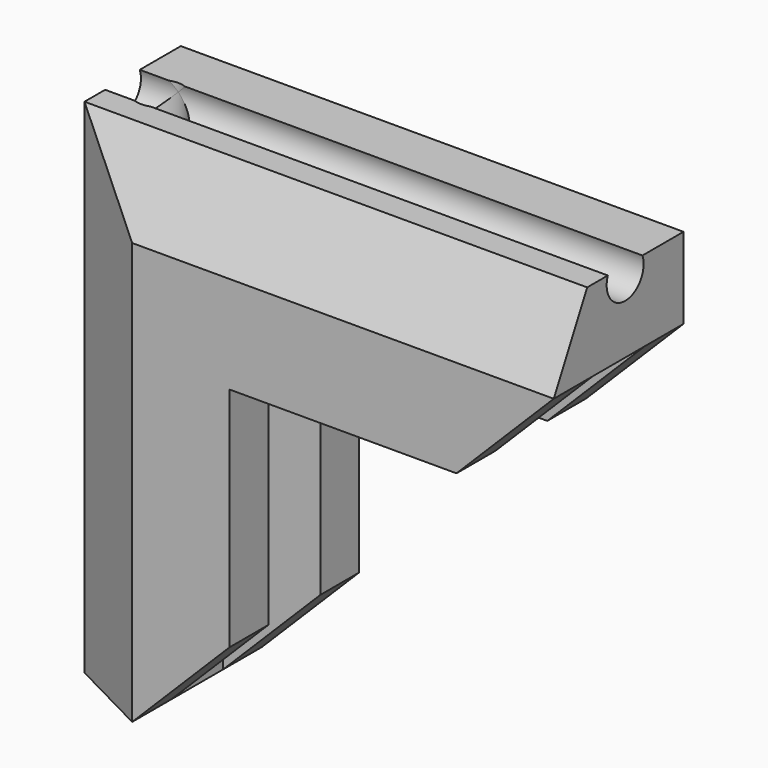
from build123d import *

# Parameters (mm, degrees)
F1_DEPTH      = 20
F2_W          = 7
F2_H          = 20
F3_DEPTH      = 2
F5_DEPTH      = 6
F6_W          = 3
F6_H          = 6
F7_DEPTH      = 25
F8_DEPTH      = 3
F12_DEPTH     = 2
F13_DEPTH     = 11
F14_T4_DEPTH  = 29
F14_T10_DEPTH = 28
F14_T17_DEPTH = 38.2867319519
F14_T24_DEPTH = 39.2867319519
F15_T1_DEPTH  = 61.1449358039
F15_T3_DEPTH  = 60.1449358039
F16_DEPTH     = 1
F17_SIZE      = 6
F20_D         = 2.85
F20_ON_F18_D  = 2.85
F22_DEPTH     = 3
F24_D         = 6.5
F24_DEPTH     = 2
F24_TIP       = 1.9527970118


# Not quite as in the source:
# - a fillet or chamfer that OpenCascade refuses, or shapes differently, is made with other operations: its cross-section is extruded or revolved along the edge and cut away or added


with BuildPart() as f1:
    # F0 (on Top) → F1 (new body)
    with BuildSketch(Plane.XY):
        Polygon((-3.1551690071, 9.1141472052), (-12.1551690071, 9.1141472052), (-12.1551690071, -0.8858527948), (-3.1551690071, -0.8858527948), (-3.1551690071, 2.1141472052), (-9.1551690071, 2.1141472052), (-9.1551690071, 6.1141472052), (-3.1551690071, 6.1141472052), align=None)
    extrude(amount=F1_DEPTH)

    # F2 (on face) → F3 (join)
    with BuildSketch(Plane(origin=(-12.1551690071, 0, 0), x_dir=(0, -1, 0), z_dir=(-1, 0, 0))):
        with Locations((-5.6141472052, 10)):
            Rectangle(F2_W, F2_H)
    extrude(amount=F3_DEPTH)

    # F4 (on face) → F5 (join)
    with BuildSketch(Plane.XY.offset(20)):
        Polygon((-12.1345976368, 9.1141472052), (-12.1551690071, 2.1141472052), (-12.1551690071, -0.8858527948), (-9.1551690071, -0.8858527948), (-9.1551690071, 2.1141472052), (-9.1551690071, 6.1141472052), (-9.1551690071, 9.1141472052), align=None)
    extrude(amount=F5_DEPTH)

    # F6 (on face) → F7 (join)
    with BuildSketch(Plane.YZ.offset(-9.1551690071)):
        with Locations((7.6141472052, 23)):
            Rectangle(F6_W, F6_H)
        with Locations((0.6141472052, 23)):
            Rectangle(F6_W, F6_H)
        Polygon((-0.8858527948, 26), (2.1141472052, 26), (6.1141472052, 26), (9.1141472052, 26), (9.1141472052, 29), (-0.8858527948, 29), align=None)
    extrude(amount=F7_DEPTH)

    # F8 (add): a face of the model
    f8_faces = [f1.faces().sort_by_distance(p)[0] for p in [
        (-10.6515768532, 4.1077318265, 26),
    ]]
    extrude(f8_faces, amount=F8_DEPTH)

    # F9: union 

    # F10: union 

    # F11 (on face) → F12 (join)
    with BuildSketch(Plane.XY.offset(29)):
        Polygon((-12.1345976368, 9.1141472052), (-12.1551690071, 2.1141472052), (15.8448309929, 2.1141472052), (15.8448309929, 9.1141472052), align=None)
    extrude(amount=F12_DEPTH)

    # F4 (on face) → F13 (join)
    with BuildSketch(Plane.XY.offset(20)):
        Polygon((-14.1551690071, 2.1141472052), (-12.1551690071, 2.1141472052), (-12.1345976368, 9.1141472052), (-14.1551690071, 9.1141472052), align=None)
    extrude(amount=F13_DEPTH)

    # F14: chamfer of 4 on 2 edges, made by hand


with BuildPart() as f14_tool2:
    # F14_s3 → F14_t4 (new body)
    with BuildSketch(Plane.XY):
        Polygon((-12.1551690071, -1.8858527948), (-16.1551690071, 2.1141472052), (-12.1551690071, 2.1141472052), align=None)
    extrude(amount=F14_T4_DEPTH)

    split(bisect_by=Plane.XZ.offset(0.8858527948), keep=Keep.BOTTOM)

    split(bisect_by=Plane.YZ.offset(-14.1551690071), keep=Keep.TOP)


with BuildPart() as f1_1:
    add(f1.part)

    # F14_t1: union F14_tool2
    add(f14_tool2.part)


with BuildPart() as f14_tool8:
    # F14_s9 → F14_t10 (new body)
    with BuildSketch(Plane.YZ.offset(-12.1551690071)):
        Polygon((-1.8858527948, 29), (2.1141472052, 33), (2.1141472052, 29), align=None)
    extrude(amount=F14_T10_DEPTH)

    split(bisect_by=Plane.XZ.offset(0.8858527948), keep=Keep.BOTTOM)

    split(bisect_by=Plane.XY.offset(31), keep=Keep.BOTTOM)


with BuildPart() as f1_2:
    add(f1_1.part)

    # F14_t7: union F14_tool8
    add(f14_tool8.part)


with BuildPart() as f14_tool15:
    # F14_s16 → F14_t17 (new body)
    with BuildSketch(Plane.YZ.offset(-22.4419009589)):
        Polygon((-1.8858527948, 29), (2.1141472052, 33), (2.1141472052, 29), align=None)
    extrude(amount=F14_T17_DEPTH)

    split(bisect_by=Plane.XZ.offset(0.8858527948), keep=Keep.BOTTOM)

    split(bisect_by=Plane.YZ.offset(-12.1551690071), keep=Keep.BOTTOM)

    split(bisect_by=Plane.YZ.offset(-14.1551690071), keep=Keep.TOP)

    split(bisect_by=Plane.XY.offset(31), keep=Keep.BOTTOM)


with BuildPart() as f14_tool22:
    # F14_s23 → F14_t24 (new body)
    with BuildSketch(Plane.XY):
        Polygon((-12.1551690071, -1.8858527948), (-16.1551690071, 2.1141472052), (-12.1551690071, 2.1141472052), align=None)
    extrude(amount=F14_T24_DEPTH)

    split(bisect_by=Plane.XZ.offset(0.8858527948), keep=Keep.BOTTOM)

    split(bisect_by=Plane.XY.offset(29), keep=Keep.TOP)

    split(bisect_by=Plane.YZ.offset(-14.1551690071), keep=Keep.TOP)

    split(bisect_by=Plane.XY.offset(31), keep=Keep.BOTTOM)


with BuildPart() as f14_tool15_1:
    add(f14_tool15.part)

    # F14_t29: intersect F14_tool22
    add(f14_tool22.part, mode=Mode.INTERSECT)


with BuildPart() as f1_3:
    add(f1_2.part)

    # F14_t13: union F14_tool15
    add(f14_tool15_1.part)

    # F15: chamfer of 4 x 6 on 2 edges, made by hand

    # F15_s2 → F15_t1 (cut)
    with BuildSketch(Plane.XY.offset(-15.5724679019)):
        Polygon((-9.1551690071, -0.8858527948), (-17.3978096942, 3.3567878923), (-13.1551690071, -0.8858527948), align=None)
    extrude(amount=F15_T1_DEPTH, mode=Mode.SUBTRACT)

    # F15_s4 → F15_t3 (cut)
    with BuildSketch(Plane.YZ.offset(-28.7276369091)):
        Polygon((-0.8858527948, 26), (3.3567878923, 34.2426406871), (-0.8858527948, 30), align=None)
    extrude(amount=F15_T3_DEPTH, mode=Mode.SUBTRACT)

    # F16 (add): a face of the model
    f16_faces = [f1_3.faces().sort_by_distance(p)[0] for p in [
        (15.8448309929, 6.2628078927, 23),
    ]]
    extrude(f16_faces, amount=F16_DEPTH)

    # F17
    f17_edges = [f1_3.edges().sort_by_distance(p)[0] for p in [
        (-3.155169, 0.614147, 0),
        (-3.155169, 7.614147, 0),
        (16.844831, 0.614147, 20),
        (16.844831, 7.614147, 20),
    ]]
    chamfer(f17_edges, length=F17_SIZE)

    # F20 (through all)
    with Locations(Plane(origin=(0, 0, 0), x_dir=(1, 0, 0), z_dir=(0, 0, -1))):
        with Locations((-11.8551690071, -4.6141472052)):
            Hole(F20_D / 2)

    # F20 on F18 (through all)
    with Locations(Plane.YZ.offset(16.8448309929)):
        with Locations((4.6141472052, 30.5)):
            Hole(F20_ON_F18_D / 2)

    # F21 (on face) → F22 (cut)
    with BuildSketch(Plane(origin=(0, 9.1141472052, 0), x_dir=(-1, 0, 0), z_dir=(0, 1, 0))):
        with BuildLine():
            Line((10.2461592647, 27.0909902577), (7.0641787494, 23.9090097423))
            ThreePointArc((7.0641787494, 23.9090097423), (9.5162067299, 23.4212710518), (10.9051690071, 25.5))
            ThreePointArc((10.9051690071, 25.5), (10.7338979552, 26.3610377228), (10.2461592647, 27.0909902577))
        make_face()
        with BuildLine():
            ThreePointArc((10.2461592647, 27.0909902577), (7.0641787494, 27.0909902577), (7.0641787494, 23.9090097423))
            Line((7.0641787494, 23.9090097423), (10.2461592647, 27.0909902577))
        make_face()
    extrude(amount=-F22_DEPTH, mode=Mode.SUBTRACT)

    # F24 (one way)
    with BuildSketch(Plane(origin=(0, 6.1141472052, 0), x_dir=(-1, 0, 0), z_dir=(0, -1, 0))):
        with Locations((8.6551690071, -25.5)):
            Circle(F24_D / 2)
    extrude(amount=-F24_DEPTH, mode=Mode.SUBTRACT)
    with Locations(Plane(origin=(0, 6.1141472052, 0), x_dir=(-1, 0, 0), z_dir=(0, -1, 0))):
        with Locations((8.6551690071, -25.5)):
            with Locations((0, 0, -(F24_DEPTH + F24_TIP / 2))):  # 118° drill point
                Cone(0, F24_D / 2, F24_TIP, mode=Mode.SUBTRACT)


solid = f1_3.part
